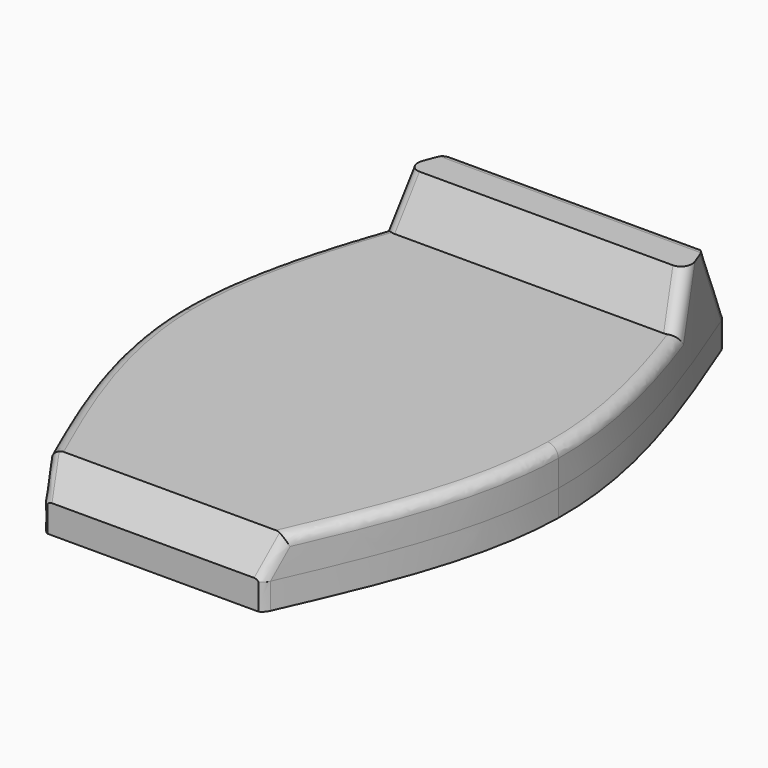
from build123d import *

# Parameters (mm, degrees)
F2_DEPTH = 10.0393754
F0_W     = 162.54427284
F0_H     = 91.0251736641
F3_DEPTH = 36.576
F4_R     = 1.27
F6_DEPTH = 3.048


# Not quite as in the source:
# - a feature names something its author has since deleted; it is built from what else it names


with BuildPart() as f2:
    # F1 (on Top) → F2 (new body)
    with BuildSketch(Plane.XY):
        with BuildLine():
            Line((22.098, 1.000200763), (0, 1.000200763))
            Line((0, 1.000200763), (0, -9.4128639907))
            Line((0, -9.4128639907), (0, -30.5107254535))
            Line((0, -30.5107254535), (12.7, -30.5107254535))
            add(Edge.make_bspline(
                [(22.098, 1.000200763), (21.9117681537, -9.8773063583), (17.3058840768, -20.1940159059), (12.7, -30.5107254535)],
                knots=[0.5153173826, 0.5153173826, 0.5153173826, 0.5153173826, 1, 1, 1, 1], degree=3))
        make_face()
        with BuildLine():
            Line((0, 36.9631461799), (0, 11.4132655167))
            Line((0, 11.4132655167), (0, 1.000200763))
            Line((0, 1.000200763), (22.098, 1.000200763))
            add(Edge.make_bspline(
                [(12.7, 36.9631461799), (17.498001392, 24.7641879428), (22.296002784, 12.5652297057), (22.098, 1.000200763)],
                knots=[0, 0, 0, 0, 0.5153173826, 0.5153173826, 0.5153173826, 0.5153173826], degree=3))
            Line((12.7, 36.9631461799), (0, 36.9631461799))
        make_face()
        with BuildLine():
            Line((0, 1.000200763), (0, 11.4132655167))
            Line((0, 11.4132655167), (0, 36.9631461799))
            Line((0, 36.9631461799), (-12.7, 36.9631461799))
            add(Edge.make_bspline(
                [(-12.7, 36.9631461799), (-17.498001392, 24.7641879428), (-22.296002784, 12.5652297057), (-22.098, 1.000200763)],
                knots=[0, 0, 0, 0, 0.5153173826, 0.5153173826, 0.5153173826, 0.5153173826], degree=3))
            Line((-22.098, 1.000200763), (0, 1.000200763))
        make_face()
        with BuildLine():
            Line((0, -9.4128639907), (0, 1.000200763))
            Line((0, 1.000200763), (-22.098, 1.000200763))
            add(Edge.make_bspline(
                [(-22.098, 1.000200763), (-21.9117681537, -9.8773063583), (-17.3058840768, -20.1940159059), (-12.7, -30.5107254535)],
                knots=[0.5153173826, 0.5153173826, 0.5153173826, 0.5153173826, 1, 1, 1, 1], degree=3))
            Line((-12.7, -30.5107254535), (0, -30.5107254535))
            Line((0, -30.5107254535), (0, -9.4128639907))
        make_face()
    extrude(amount=F2_DEPTH)

    # F0 (on Right) → F3 (cut, symmetric)
    with BuildSketch(Plane.YZ):
        with Locations((14.1260512173, 4.4935680926)):
            Rectangle(F0_W, F0_H)
        Polygon((3.2016009947, 0), (-30.665065672, 0), (-28.0743391016, 4.3514131215), (-17.965065672, 4.3514131215), (3.2016009947, 4.3514131215), (24.3682676614, 4.3514131215), (26.8577352928, 10.0393698853), (31.0910686261, 10.0393698853), (37.0682676614, 0), align=None, mode=Mode.SUBTRACT)
    extrude(amount=F3_DEPTH, both=True, mode=Mode.SUBTRACT)

    # F4
    f4_edges = [f2.edges().sort_by_distance(p)[0] for p in [
        (-21.914013, -2.246239, 4.351413),
        (-17.021737, 25.613292, 7.196056),
        (17.021737, 25.613292, 7.196056),
        (21.914013, -2.246239, 4.351413),
        (-13.852046, 34.027829, 5.106754),
        (13.852046, 34.027829, 5.106754),
        (0, 31.091069, 10.03937),
        (13.243552, -29.292588, 2.305229),
        (-13.243552, -29.292588, 2.305229),
    ]]
    fillet(f4_edges, radius=F4_R)

    # F6 (add): a face of the model
    f6_faces = [f2.faces().sort_by_distance(p)[0] for p in [
        (0, 3.0480549661, 0),
    ]]
    extrude(f6_faces, amount=F6_DEPTH)


solid = f2.part
